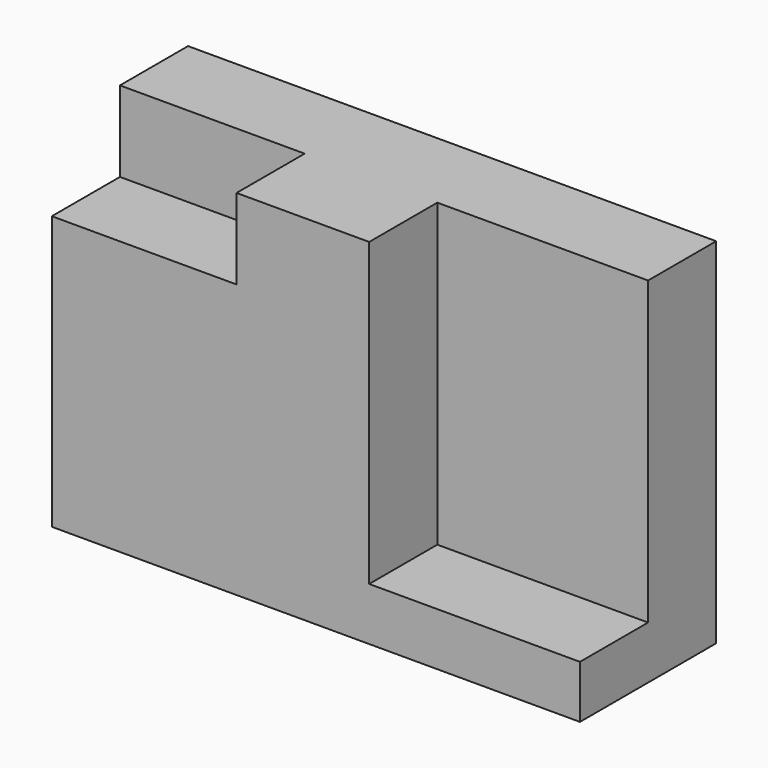
from build123d import *

# Parameters (mm, degrees)
F0_W     = 157.5917825103
F0_H     = 105.6277751923
F1_DEPTH = 50.8
F2_W     = 55.120697245
F2_H     = 24.0394249558
F3_DEPTH = 25.4
F2_W_2   = 62.8910250962
F2_H_2   = 89.8443162441
F4_DEPTH = 25.4


with BuildPart() as f1:
    # F0 (on Front) → F1 (new body)
    with BuildSketch(Plane.XZ):
        with Locations((2.6710517704, 2.549637109)):
            Rectangle(F0_W, F0_H)
    extrude(amount=F1_DEPTH)

    # F2 (on face) → F3 (cut)
    with BuildSketch(Plane.XZ.offset(50.8)):
        with Locations((-48.5644908622, 43.3438122272)):
            Rectangle(F2_W, F2_H)
    extrude(amount=-F3_DEPTH, mode=Mode.SUBTRACT)

    # F2 (on face) → F4 (cut)
    with BuildSketch(Plane.XZ.offset(50.8)):
        with Locations((50.0214304775, 10.4413665831)):
            Rectangle(F2_W_2, F2_H_2)
    extrude(amount=-F4_DEPTH, mode=Mode.SUBTRACT)


solid = f1.part
